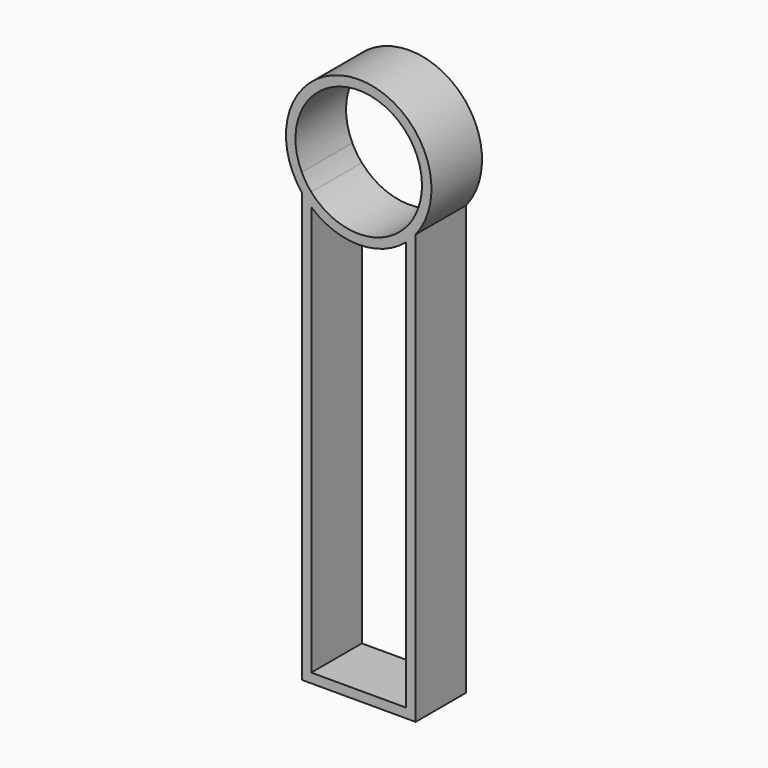
from build123d import *

# Parameters (mm, degrees)
F1_DEPTH = 20


# Not quite as in the source:
# - a feature names something its author has since deleted; it is built from what else it names


with BuildPart() as f1:
    # F0 (on Front) → F1 (new body)
    with BuildSketch(Plane.XZ):
        with BuildLine():
            ThreePointArc((-18, 68.354232338), (-4.472135955, 96.5656189147), (20, 77.072030225))
            ThreePointArc((20, 77.072030225), (19.4935886896, 72.59989427), (18, 68.354232338))
            Line((18, 68.354232338), (18, 62.7542091618))
            ThreePointArc((18, 62.7542091618), (21.7140507506, 69.489154781), (23, 77.072030225))
            ThreePointArc((23, 77.072030225), (-7.5828754441, 98.7860809757), (-18, 62.7542091618))
            Line((-18, 62.7542091618), (-18, 68.354232338))
        make_face()
        with BuildLine():
            ThreePointArc((-15, 63.8432736697), (-16.6534436987, 65.9967057163), (-18, 68.354232338))
            Line((-18, 68.354232338), (-18, 62.7542091618))
            ThreePointArc((-18, 62.7542091618), (-16.5734766958, 61.1246207109), (-15, 59.6364344509))
            Line((-15, 59.6364344509), (-15, 63.8432736697))
        make_face()
        with BuildLine():
            Line((18, 62.7542091618), (18, 68.354232338))
            ThreePointArc((18, 68.354232338), (16.6534436987, 65.9967057163), (15, 63.8432736697))
            Line((15, 63.8432736697), (15, 59.6364344509))
            ThreePointArc((15, 59.6364344509), (16.5734766958, 61.1246207109), (18, 62.7542091618))
        make_face()
        with BuildLine():
            ThreePointArc((15, 63.8432736697), (0, 57.072030225), (-15, 63.8432736697))
            Line((-15, 63.8432736697), (-15, 59.6364344509))
            ThreePointArc((-15, 59.6364344509), (0, 54.072030225), (15, 59.6364344509))
            Line((15, 59.6364344509), (15, 63.8432736697))
        make_face()
        with BuildLine():
            ThreePointArc((-15, 59.6364344509), (-16.5734766958, 61.1246207109), (-18, 62.7542091618))
            Line((-18, 62.7542091618), (-18, -72.927969775))
            Line((-18, -72.927969775), (18, -72.927969775))
            Line((18, -72.927969775), (18, 62.7542091618))
            ThreePointArc((18, 62.7542091618), (16.5734766958, 61.1246207109), (15, 59.6364344509))
            Line((15, 59.6364344509), (15, -69.927969775))
            Line((15, -69.927969775), (-15, -69.927969775))
            Line((-15, -69.927969775), (-15, 59.6364344509))
        make_face()
    extrude(amount=F1_DEPTH)


solid = f1.part
